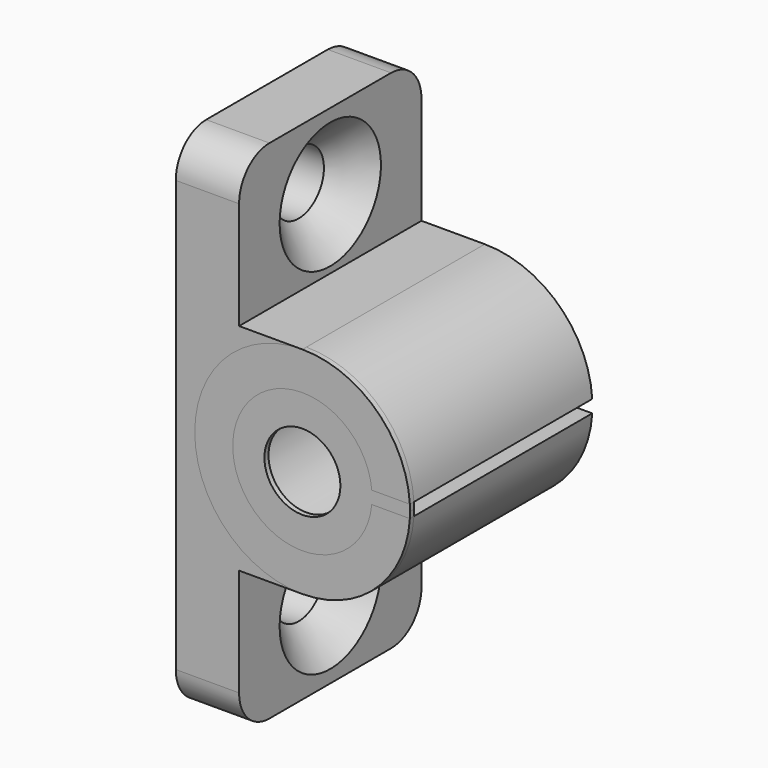
from build123d import *
from build123d import SkipClean  # not in build123d's __all__

# Parameters (mm, degrees)
F1_DEPTH       = 18
F2_R           = 5.5
F3_DEPTH       = 18
F5_D           = 5
F5_CSINK_D     = 10
F5_CSINK_ANGLE = 90
F6_W           = 7.3579490118
F6_H           = 1
F7_DEPTH       = 18
F8_R           = 3
F9_R           = 8.5
F9_R_2         = 3
F10_DEPTH      = 0.4


with BuildPart() as f1:
    # F0 (on Front) → F1 (new body)
    with BuildSketch(Plane.XZ):
        with BuildLine():
            ThreePointArc((-5, -6.8738635424), (-8.5, 0), (-5, 6.8738635424))
            Line((-5, 6.8738635424), (-5, 8.5))
            Line((-5, 8.5), (-5, 20))
            Line((-5, 20), (-10, 20))
            Line((-10, 20), (-10, -20))
            Line((-10, -20), (-5, -20))
            Line((-5, -20), (-5, -8.5))
            Line((-5, -8.5), (-5, -6.8738635424))
        make_face()
        with BuildLine():
            ThreePointArc((0, -8.5), (6.0104076401, -6.0104076401), (8.5, 0))
            ThreePointArc((8.5, 0), (6.0104076401, 6.0104076401), (0, 8.5))
            ThreePointArc((0, 8.5), (-2.6288932927, 8.0832493501), (-5, 6.8738635424))
            Line((-5, 6.8738635424), (-5, -6.8738635424))
            ThreePointArc((-5, -6.8738635424), (-2.6288932927, -8.0832493501), (0, -8.5))
        make_face()
        with BuildLine():
            Line((-5, -8.5), (0, -8.5))
            ThreePointArc((0, -8.5), (-2.6288932927, -8.0832493501), (-5, -6.8738635424))
            Line((-5, -6.8738635424), (-5, -8.5))
        make_face()
        with BuildLine():
            Line((-5, -6.8738635424), (-5, 6.8738635424))
            ThreePointArc((-5, 6.8738635424), (-8.5, 0), (-5, -6.8738635424))
        make_face()
        with BuildLine():
            ThreePointArc((-5, 6.8738635424), (-2.6288932927, 8.0832493501), (0, 8.5))
            Line((0, 8.5), (-5, 8.5))
            Line((-5, 8.5), (-5, 6.8738635424))
        make_face()
    extrude(amount=F1_DEPTH)

    # F2 (on face) → F3 (cut, through all)
    with BuildSketch(Plane.XZ.offset(18)):
        Circle(F2_R)
    extrude(amount=-F3_DEPTH, mode=Mode.SUBTRACT)

    # F5 (through all)
    with Locations(Plane.YZ.offset(-5)):
        with Locations((-9, -14), (-9, 14)):
            CounterSinkHole(F5_D / 2, F5_CSINK_D / 2, counter_sink_angle=F5_CSINK_ANGLE)

    # F6 (on Front) → F7 (cut, through all)
    with BuildSketch(Plane.XZ):
        with Locations((7.1057528257, 0)):
            Rectangle(F6_W, F6_H)
    extrude(amount=F7_DEPTH, mode=Mode.SUBTRACT)

    # F8
    f8_edges = [f1.edges().sort_by_distance(p)[0] for p in [
        (-7.5, -18, -20),
        (-7.5, -18, 20),
        (-7.5, 0, 20),
        (-7.5, 0, -20),
    ]]
    fillet(f8_edges, radius=F8_R)

    # F9 (on face) → F10 (join)
    with BuildSketch(Plane.XZ.offset(18)):
        Circle(F9_R)
        Circle(F9_R_2, mode=Mode.SUBTRACT)
    with SkipClean():  # cleaning this boolean's faces spoils the solid; the shape is the same uncleaned
        extrude(amount=-F10_DEPTH)


solid = f1.part
